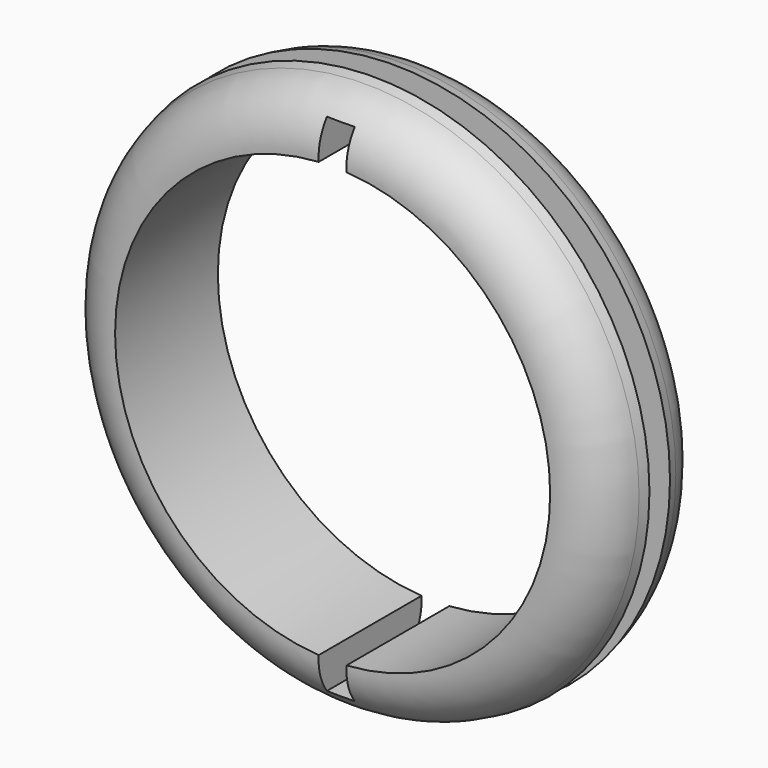
from build123d import *

# Parameters (mm, degrees)
F4_W          = 1.0840747273
F4_H          = 19.680833444
F5_DEPTH      = 25
F5_DEPTH_BACK = 25


# Not quite as in the source:
# - a fillet or chamfer that OpenCascade refuses, or shapes differently, is made with other operations: its cross-section is extruded or revolved along the edge and cut away or added


with BuildPart() as f2:
    # F2: sweep along a path in F0
    with BuildLine(Plane.XZ) as f2_path:
        CenterArc((0, 0), 8.65, 0, 360)
    # F1 (on Right) → F2 (sweep)
    with BuildSketch(Plane.YZ):
        Polygon((-2.5, 8.4675319269), (0, 8.4675319269), (2.5, 8.4675319269), (2.6424242295, 10.246030055), (0.5, 10.7327634469), (0.5, 9.5877971399), (0.344154765, 9.4675319269), (0, 9.4675319269), (-0.344154765, 9.4675319269), (-0.5, 9.5877971399), (-0.5, 10.7327634469), (-2.6424242295, 10.246030055), align=None)
    sweep(path=f2_path.line)

    # F3: fillet of radius 2.0708896165 on 2 edges, made by hand

    # F3_s1 → F3_t2 (revolve, cut)
    with BuildSketch(Plane.XY):
        with BuildLine():
            ThreePointArc((8.4585593646, -2.4992814666), (9.85018085, -2.103755641), (10.6432988419, -0.8937908116))
            Line((10.6432988419, -0.8937908116), (10.246030055, -2.6424242295))
            Line((10.246030055, -2.6424242295), (8.4585593646, -2.4992814666))
        make_face()
    revolve(axis=Axis((0, -2.6424242295, 0), (0, -1, 0)), mode=Mode.SUBTRACT)

    # F3_s3 → F3_t4 (revolve, cut)
    with BuildSketch(Plane.XY):
        with BuildLine():
            ThreePointArc((8.4585593646, 2.4992814666), (9.85018085, 2.103755641), (10.6432988419, 0.8937908116))
            Line((10.6432988419, 0.8937908116), (10.246030055, 2.6424242295))
            Line((10.246030055, 2.6424242295), (8.4585593646, 2.4992814666))
        make_face()
    revolve(axis=Axis((0, 2.6424242295, 0), (0, -1, 0)), mode=Mode.SUBTRACT)

    # F4 (on Front) → F5 (cut, two sides)
    with BuildSketch(Plane.XZ) as f5_sk:
        Rectangle(F4_W, F4_H)
    extrude(amount=-F5_DEPTH, mode=Mode.SUBTRACT)
    extrude(f5_sk.sketch, amount=F5_DEPTH_BACK, mode=Mode.SUBTRACT)


solid = f2.part
